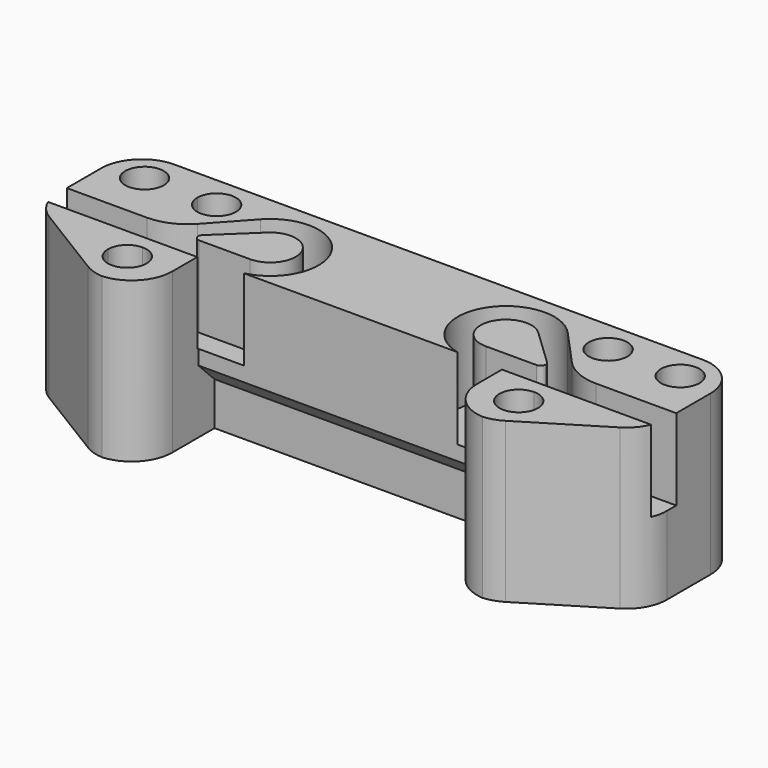
from build123d import *

# Parameters (mm, degrees)
F1_DEPTH    = 15.7
F2_W        = 10.0960650777
F2_H        = 2.7
F3_DEPTH    = 8
F4_R        = 5
F5_T1_DEPTH = 26.8923143391
F5_T3_DEPTH = 21.3473434867
F5_T5_DEPTH = 35.7
F6_W        = 15
F6_H        = 6.25
F7_DEPTH    = 2
F8_SIZE     = 1.99999


# Not quite as in the source:
# - a fillet or chamfer that OpenCascade refuses, or shapes differently, is made with other operations: its cross-section is extruded or revolved along the edge and cut away or added
# - a fillet or chamfer is up to 0.001 mm smaller than in the source, because OpenCascade refuses the exact size


with BuildPart() as f1:
    # F0 (on Top) → F1 (new body)
    with BuildSketch(Plane.XY):
        Polygon((30, 9), (0, 9), (0, -1.8), (15, -1.8), (15, -9), (19.5954625243, -9), (30, -2.6151265483), align=None)
        with BuildLine():
            ThreePointArc((21.17, -5.2), (17.9264971157, -6.5435028843), (19.27, -3.3))
            ThreePointArc((19.27, -3.3), (20.6135028843, -3.8564971157), (21.17, -5.2))
        make_face(mode=Mode.SUBTRACT)
        with BuildLine():
            ThreePointArc((19.27, 3.9), (17.9264971157, 7.1435028843), (21.17, 5.8))
            ThreePointArc((21.17, 5.8), (20.6135028843, 4.4564971157), (19.27, 3.9))
        make_face(mode=Mode.SUBTRACT)
        with BuildLine():
            ThreePointArc((24.47, 5.8), (26.37, 7.7), (28.27, 5.8))
            ThreePointArc((28.27, 5.8), (26.37, 3.9), (24.47, 5.8))
        make_face(mode=Mode.SUBTRACT)
    extrude(amount=F1_DEPTH)

    # F2 (on face) → F3 (cut)
    with BuildSketch(Plane.XY.offset(15.7)):
        with BuildLine():
            ThreePointArc((11.6039349223, 0.3250306588), (9.2827431951, 3.7535073497), (13.3280728534, 4.6353754864))
            Line((13.3280728534, 4.6353754864), (16.2527744297, 1.8499454137))
            ThreePointArc((16.2527744297, 1.8499454137), (16.328577113, 2.3348713274), (16.3539349223, 2.8250306588))
            ThreePointArc((16.3539349223, 2.8250306588), (16.0328522645, 4.5417691876), (15.1130123218, 6.0264172029))
            ThreePointArc((15.1130123218, 6.0264172029), (7.5069370658, 5.2285923001), (10.5215341623, -1.8))
            Line((10.5215341623, -1.8), (12.6863356823, -1.8))
            ThreePointArc((12.6863356823, -1.8), (14.376262754, -1.0320016711), (15.6428085277, 0.3250306588))
            Line((15.6428085277, 0.3250306588), (11.6039349223, 0.3250306588))
        make_face()
        with BuildLine():
            ThreePointArc((16.3539349223, 2.8250306588), (16.328577113, 2.3348713274), (16.2527744297, 1.8499454137))
            Line((16.2527744297, 1.8499454137), (16.9487625085, 1.1870996243))
            ThreePointArc((16.9487625085, 1.1870996243), (17.0635074373, 1.0219903081), (17.1039349223, 0.8250306588))
            ThreePointArc((17.1039349223, 0.8250306588), (16.9574883129, 0.4714772682), (16.6039349223, 0.3250306588))
            Line((16.6039349223, 0.3250306588), (15.6428085277, 0.3250306588))
            ThreePointArc((15.6428085277, 0.3250306588), (14.376262754, -1.0320016711), (12.6863356823, -1.8))
            Line((12.6863356823, -1.8), (15, -1.8))
            Line((15, -1.8), (15, -1.9249693412))
            Line((15, -1.9249693412), (19.9039349223, -1.9249693412))
            Line((19.9039349223, -1.9249693412), (19.9039349223, 0.7750306588))
            Line((19.9039349223, 0.7750306588), (15.1130123218, 6.0264172029))
            ThreePointArc((15.1130123218, 6.0264172029), (16.0328522645, 4.5417691876), (16.3539349223, 2.8250306588))
        make_face()
        with Locations((24.9519674612, -0.5749693412)):
            Rectangle(F2_W, F2_H)
    extrude(amount=-F3_DEPTH, mode=Mode.SUBTRACT)

    # F4
    f4_edges = [f1.edges().sort_by_distance(p)[0] for p in [
        (19.903935, 0.775031, 11.7),
    ]]
    fillet(f4_edges, radius=F4_R)

    # F5: fillet of radius 4 on 4 edges, made by hand

    # F5_s2 → F5_t1 (cut)
    with BuildSketch(Plane.XY.offset(-5.5961571696)):
        with BuildLine():
            ThreePointArc((30, -0.3766636805), (29.4905957559, -2.3300559271), (28.0921293656, -3.7859150232))
            Line((28.0921293656, -3.7859150232), (30, -2.6151265483))
            Line((30, -2.6151265483), (30, -0.3766636805))
        make_face()
    extrude(amount=F5_T1_DEPTH, mode=Mode.SUBTRACT)

    # F5_s4 → F5_t3 (cut)
    with BuildSketch(Plane.XY.offset(-2.8236717433)):
        with BuildLine():
            ThreePointArc((20.5581231925, -8.4092513427), (19.5529608525, -8.8494808332), (18.465993827, -9))
            Line((18.465993827, -9), (19.5954625243, -9))
            Line((19.5954625243, -9), (20.5581231925, -8.4092513427))
        make_face()
    extrude(amount=F5_T3_DEPTH, mode=Mode.SUBTRACT)

    # F5_s6 → F5_t5 (cut)
    with BuildSketch(Plane.XY.offset(-10)):
        with BuildLine():
            ThreePointArc((15, -5), (16.1715728753, -7.8284271247), (19, -9))
            Line((19, -9), (15, -9))
            Line((15, -9), (15, -5))
        make_face()
        with BuildLine():
            ThreePointArc((30, 5), (28.8284271247, 7.8284271247), (26, 9))
            Line((26, 9), (30, 9))
            Line((30, 9), (30, 5))
        make_face()
    extrude(amount=F5_T5_DEPTH, mode=Mode.SUBTRACT)

    # F6 (on face) → F7 (cut)
    with BuildSketch(Plane.XZ.offset(1.8)):
        with Locations((7.5, 3.125)):
            Rectangle(F6_W, F6_H)
    extrude(amount=-F7_DEPTH, mode=Mode.SUBTRACT)

    # F8 (size 2 in the source; OpenCascade refuses exactly that, so slightly less here)
    f8_edges = [f1.edges().sort_by_distance(p)[0] for p in [
        (7.5, 0.2, 6.25),
    ]]
    chamfer(f8_edges, length=F8_SIZE)

    # F9: F1 across plane


with BuildPart() as f1_1:
    add(f1.part)
    add(f1.part.mirror(Plane.YZ))


solid = f1_1.part
